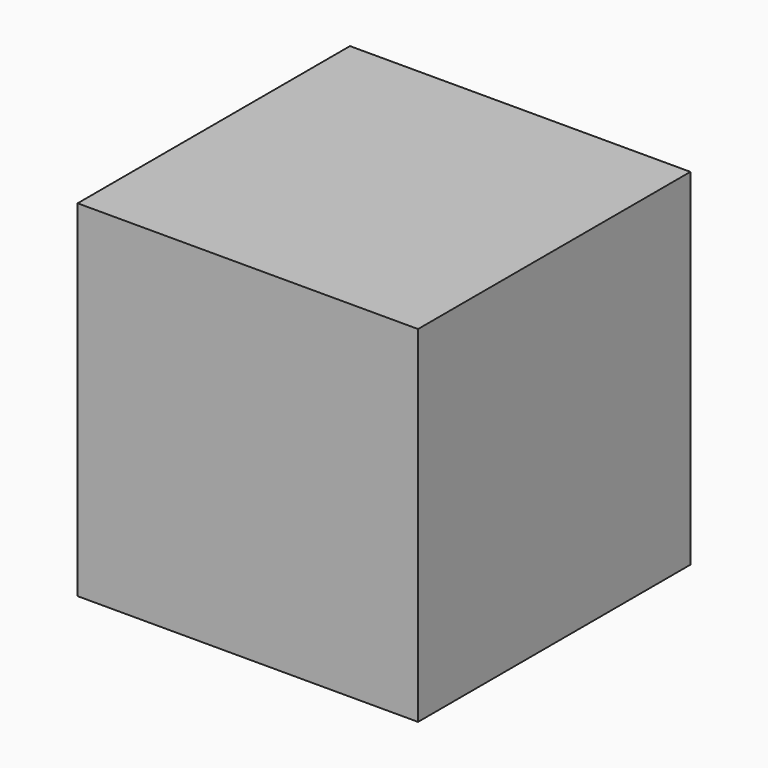
from build123d import *

# Parameters (mm, degrees)
F0_W     = 25
F0_H     = 25
F1_DEPTH = 25.4
F4_DEPTH = 25


# Not quite as in the source:
# - the program builds the solid bodies; features that only make, move or delete a surface that nothing else refers to are left out


with BuildPart() as f1:
    # F0 (on Top) → F1 (new body)
    with BuildSketch(Plane.XY):
        Rectangle(F0_W, F0_H)
    extrude(amount=F1_DEPTH)

    # F0 (on Top) → F4 (join)
    with BuildSketch(Plane.XY):
        Rectangle(F0_W, F0_H)
    extrude(amount=F4_DEPTH)


solid = f1.part
